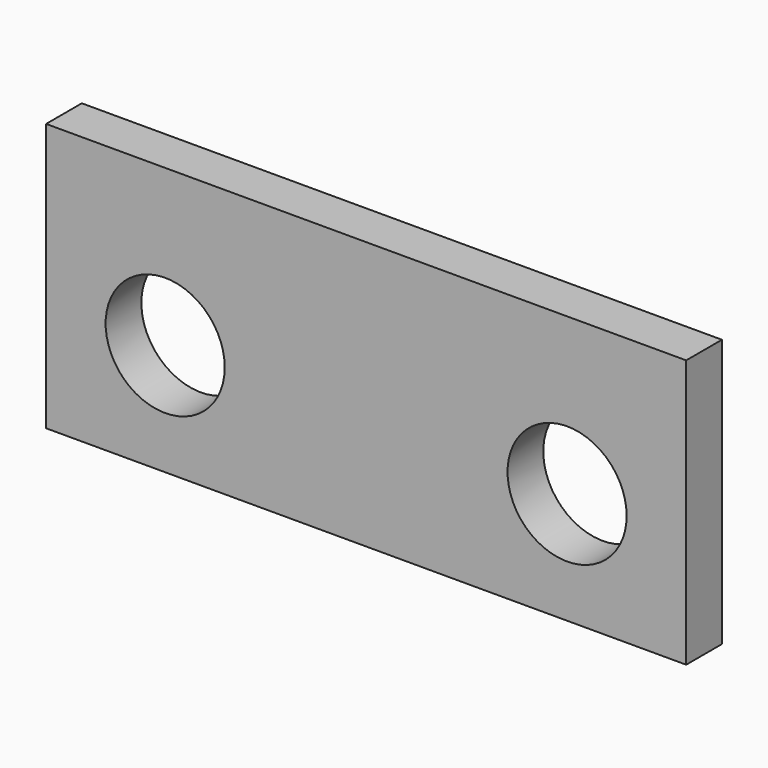
from build123d import *

# Parameters (mm, degrees)
F0_W     = 273.05
F0_H     = 114.3
F1_DEPTH = 19.05
F2_R     = 25.4
F3_DEPTH = 25.4


# Not quite as in the source:
# - a feature names something its author has since deleted; it is built from what else it names


with BuildPart() as f1:
    # F0 (on Front) → F1 (new body)
    with BuildSketch(Plane.XZ):
        with Locations((136.525, 57.15)):
            Rectangle(F0_W, F0_H)
    extrude(amount=F1_DEPTH)

    # F2 (on face) → F3 (cut)
    with BuildSketch(Plane.XZ.offset(19.05)):
        with Locations((50.8, 47.625)):
            Circle(F2_R)
        with Locations((222.25, 47.625)):
            Circle(F2_R)
    extrude(amount=-F3_DEPTH, mode=Mode.SUBTRACT)


solid = f1.part
